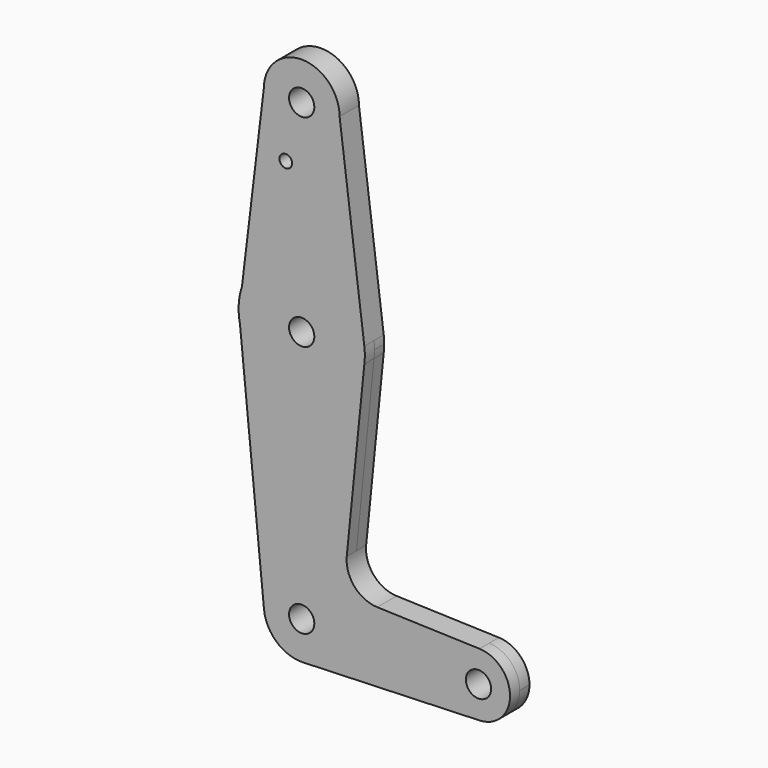
from build123d import *

# Parameters (mm, degrees)
F0_R        = 3.175
F0_R_2      = 1.5875
F1_DEPTH    = 3.048
F1_FACE_R   = 3.175
F1_FACE_R_2 = 1.5875
F2_DEPTH    = 3.048


# Not quite as in the source:
# - after a boolean that leaves OpenCascade's solid faulty, fix() repairs it


with BuildPart() as f1:
    # F0 (on Front) → F1 (new body)
    with BuildSketch(Plane.XZ):
        with BuildLine():
            ThreePointArc((-53.975, 50.4670464277), (-44.45, 40.9420464277), (-34.925, 50.4670464277))
            ThreePointArc((-34.925, 50.4670464277), (-44.45, 59.9920464277), (-53.975, 50.4670464277))
        make_face()
        with Locations((-44.45, 50.4670464277)):
            Circle(F0_R, mode=Mode.SUBTRACT)
        with BuildLine():
            Line((-28.7025430953, 1.6753357581), (-34.925, 50.4670464277))
            ThreePointArc((-34.925, 50.4670464277), (-44.45, 40.9420464277), (-53.975, 50.4670464277))
            Line((-53.975, 50.4670464277), (-59.4731707335, 4.7973452602))
            ThreePointArc((-59.4731707335, 4.7973452602), (-42.8475383164, 15.4609611278), (-28.7025430953, 1.6753357581))
        make_face()
        with Locations((-48.45572263, 36.1922464277)):
            Circle(F0_R_2, mode=Mode.SUBTRACT)
        with BuildLine():
            ThreePointArc((-28.575, -0.3329535723), (-28.6069178604, 0.6732140673), (-28.7025430953, 1.6753357581))
            ThreePointArc((-28.7025430953, 1.6753357581), (-42.8475383164, 15.4609611278), (-59.4731707335, 4.7973452602))
            ThreePointArc((-59.4731707335, 4.7973452602), (-60.0824637934, 2.4314090575), (-60.3215080228, 0))
            Line((-60.3215080228, 0), (-59.9501789354, -3.7622505804))
            ThreePointArc((-59.9501789354, -3.7622505804), (-43.7288188136, -16.1915639369), (-28.7025430953, -2.3412429026))
            ThreePointArc((-28.7025430953, -2.3412429026), (-28.6069178604, -1.3391212118), (-28.575, -0.3329535723))
        make_face()
        with Locations((-44.45, -0.3329535723)):
            Circle(F0_R, mode=Mode.SUBTRACT)
        with BuildLine():
            Line((-59.9501789354, -3.7622505804), (-60.3215080228, 0))
            ThreePointArc((-60.3215080228, 0), (-60.2482378134, -1.8922184603), (-59.9501789354, -3.7622505804))
        make_face()
        with BuildLine():
            Line((-33.1183182382, -46.317436026), (-28.7025430953, -2.3412429026))
            ThreePointArc((-28.7025430953, -2.3412429026), (-43.7288188136, -16.1915639369), (-59.9501789354, -3.7622505804))
            Line((-59.9501789354, -3.7622505804), (-53.928942688, -64.7685125051))
            ThreePointArc((-53.928942688, -64.7685125051), (-44.9183459706, -54.3194748683), (-34.925, -63.8329535723))
            ThreePointArc((-34.925, -63.8329535723), (-37.4756032752, -70.3201267105), (-43.7614126668, -73.3330310711))
            Line((-43.7614126668, -73.3330310711), (0.2823318858, -71.7654307992))
            ThreePointArc((0.2823318858, -71.7654307992), (-7.9374918809, -63.8443065466), (0.2596391732, -55.8997011655))
            Line((0.2596391732, -55.8997011655), (-25.4679521782, -55.0576895661))
            ThreePointArc((-25.4679521782, -55.0576895661), (-31.1901358295, -52.3480122444), (-33.1183182382, -46.317436026))
        make_face()
        with BuildLine():
            ThreePointArc((-34.925, -63.8329535723), (-44.9183459706, -54.3194748683), (-53.928942688, -64.7685125051))
            ThreePointArc((-53.928942688, -64.7685125051), (-50.8501155234, -70.8873242945), (-44.4614490432, -73.3579466914))
            Line((-44.4614490432, -73.3579466914), (-43.7614126668, -73.3330310711))
            ThreePointArc((-43.7614126668, -73.3330310711), (-37.4756032752, -70.3201267105), (-34.925, -63.8329535723))
        make_face()
        with Locations((-44.45, -63.8329535723)):
            Circle(F0_R, mode=Mode.SUBTRACT)
        with BuildLine():
            Line((-43.7614126668, -73.3330310711), (-44.4614490432, -73.3579466914))
            ThreePointArc((-44.4614490432, -73.3579466914), (-44.111201737, -73.3519262446), (-43.7614126668, -73.3330310711))
        make_face()
        with BuildLine():
            ThreePointArc((7.9375, -63.8329535723), (5.7037177432, -58.3128530156), (0.2596391732, -55.8997011655))
            ThreePointArc((0.2596391732, -55.8997011655), (-7.9374918809, -63.8443065466), (0.2823318858, -71.7654307992))
            ThreePointArc((0.2823318858, -71.7654307992), (5.7116072866, -69.344890478), (7.9375, -63.8329535723))
        make_face()
        with Locations((0, -63.8329535723)):
            Circle(F0_R, mode=Mode.SUBTRACT)
    extrude(amount=F1_DEPTH)

    # F0 (on Front) + F1_face (on face) → F2 (join)
    with BuildSketch(Plane.XZ):
        with BuildLine():
            ThreePointArc((-53.975, 50.4670464277), (-44.45, 40.9420464277), (-34.925, 50.4670464277))
            ThreePointArc((-34.925, 50.4670464277), (-44.45, 59.9920464277), (-53.975, 50.4670464277))
        make_face()
        with Locations((-44.45, 50.4670464277)):
            Circle(F0_R, mode=Mode.SUBTRACT)
        with BuildLine():
            Line((-28.7025430953, 1.6753357581), (-34.925, 50.4670464277))
            ThreePointArc((-34.925, 50.4670464277), (-44.45, 40.9420464277), (-53.975, 50.4670464277))
            Line((-53.975, 50.4670464277), (-59.4731707335, 4.7973452602))
            ThreePointArc((-59.4731707335, 4.7973452602), (-42.8475383164, 15.4609611278), (-28.7025430953, 1.6753357581))
        make_face()
        with Locations((-48.45572263, 36.1922464277)):
            Circle(F0_R_2, mode=Mode.SUBTRACT)
        with BuildLine():
            ThreePointArc((-28.575, -0.3329535723), (-28.6069178604, 0.6732140673), (-28.7025430953, 1.6753357581))
            ThreePointArc((-28.7025430953, 1.6753357581), (-42.8475383164, 15.4609611278), (-59.4731707335, 4.7973452602))
            ThreePointArc((-59.4731707335, 4.7973452602), (-60.0824637934, 2.4314090575), (-60.3215080228, 0))
            Line((-60.3215080228, 0), (-59.9501789354, -3.7622505804))
            ThreePointArc((-59.9501789354, -3.7622505804), (-43.7288188136, -16.1915639369), (-28.7025430953, -2.3412429026))
            ThreePointArc((-28.7025430953, -2.3412429026), (-28.6069178604, -1.3391212118), (-28.575, -0.3329535723))
        make_face()
        with Locations((-44.45, -0.3329535723)):
            Circle(F0_R, mode=Mode.SUBTRACT)
        with BuildLine():
            Line((-59.9501789354, -3.7622505804), (-60.3215080228, 0))
            ThreePointArc((-60.3215080228, 0), (-60.2482378134, -1.8922184603), (-59.9501789354, -3.7622505804))
        make_face()
        with BuildLine():
            Line((-33.1183182382, -46.317436026), (-28.7025430953, -2.3412429026))
            ThreePointArc((-28.7025430953, -2.3412429026), (-43.7288188136, -16.1915639369), (-59.9501789354, -3.7622505804))
            Line((-59.9501789354, -3.7622505804), (-53.928942688, -64.7685125051))
            ThreePointArc((-53.928942688, -64.7685125051), (-44.9183459706, -54.3194748683), (-34.925, -63.8329535723))
            ThreePointArc((-34.925, -63.8329535723), (-37.4756032752, -70.3201267105), (-43.7614126668, -73.3330310711))
            Line((-43.7614126668, -73.3330310711), (0.2823318858, -71.7654307992))
            ThreePointArc((0.2823318858, -71.7654307992), (-7.9374918809, -63.8443065466), (0.2596391732, -55.8997011655))
            Line((0.2596391732, -55.8997011655), (-25.4679521782, -55.0576895661))
            ThreePointArc((-25.4679521782, -55.0576895661), (-31.1901358295, -52.3480122444), (-33.1183182382, -46.317436026))
        make_face()
        with BuildLine():
            ThreePointArc((-34.925, -63.8329535723), (-44.9183459706, -54.3194748683), (-53.928942688, -64.7685125051))
            ThreePointArc((-53.928942688, -64.7685125051), (-50.8501155234, -70.8873242945), (-44.4614490432, -73.3579466914))
            Line((-44.4614490432, -73.3579466914), (-43.7614126668, -73.3330310711))
            ThreePointArc((-43.7614126668, -73.3330310711), (-37.4756032752, -70.3201267105), (-34.925, -63.8329535723))
        make_face()
        with Locations((-44.45, -63.8329535723)):
            Circle(F0_R, mode=Mode.SUBTRACT)
        with BuildLine():
            Line((-43.7614126668, -73.3330310711), (-44.4614490432, -73.3579466914))
            ThreePointArc((-44.4614490432, -73.3579466914), (-44.111201737, -73.3519262446), (-43.7614126668, -73.3330310711))
        make_face()
        with BuildLine():
            ThreePointArc((7.9375, -63.8329535723), (5.7037177432, -58.3128530156), (0.2596391732, -55.8997011655))
            ThreePointArc((0.2596391732, -55.8997011655), (-7.9374918809, -63.8443065466), (0.2823318858, -71.7654307992))
            ThreePointArc((0.2823318858, -71.7654307992), (5.7116072866, -69.344890478), (7.9375, -63.8329535723))
        make_face()
        with Locations((0, -63.8329535723)):
            Circle(F0_R, mode=Mode.SUBTRACT)
    with BuildSketch(Plane(origin=(-39.2541813262, -3.048, -16.9379503901), x_dir=(1, 0, 0), z_dir=(0, -1, 0))):
        with BuildLine():
            ThreePointArc((4.3291813262, 67.4049968178), (-5.1958186738, 76.9299968178), (-14.7208186738, 67.4049968178))
            Line((-14.7208186738, 67.4049968178), (-20.2189894074, 21.7352956503))
            ThreePointArc((-20.2189894074, 21.7352956503), (-21.0462252614, 17.4883065075), (-20.6959976093, 13.1756998097))
            Line((-20.6959976093, 13.1756998097), (-14.6747613619, -47.830562115))
            ThreePointArc((-14.6747613619, -47.830562115), (-11.3322126787, -54.1799392572), (-4.5072313406, -56.395080681))
            Line((-4.5072313406, -56.395080681), (39.536513212, -54.8274804091))
            ThreePointArc((39.536513212, -54.8274804091), (47.1916732071, -46.8836502078), (39.5138204994, -38.9617507754))
            Line((39.5138204994, -38.9617507754), (13.7862291479, -38.119739176))
            ThreePointArc((13.7862291479, -38.119739176), (8.0640454966, -35.4100618543), (6.1358630879, -29.3794856359))
            Line((6.1358630879, -29.3794856359), (10.5516382309, 14.5967074875))
            ThreePointArc((10.5516382309, 14.5967074875), (10.6791813262, 16.6049968178), (10.5516382309, 18.6132861482))
            Line((10.5516382309, 18.6132861482), (4.3291813262, 67.4049968178))
        make_face()
        with Locations((-5.1958186738, 67.4049968178)):
            Circle(F1_FACE_R, mode=Mode.SUBTRACT)
        with Locations((-9.2015413039, 53.1301968178)):
            Circle(F1_FACE_R_2, mode=Mode.SUBTRACT)
        with Locations((-5.1958186738, 16.6049968178)):
            Circle(F1_FACE_R, mode=Mode.SUBTRACT)
        with Locations((-5.1958186738, -46.8950031822)):
            Circle(F1_FACE_R, mode=Mode.SUBTRACT)
        with Locations((39.2541813262, -46.8950031822)):
            Circle(F1_FACE_R, mode=Mode.SUBTRACT)
    extrude(amount=F2_DEPTH)

    add(f1.part.fix(), mode=Mode.REPLACE)


solid = f1.part
